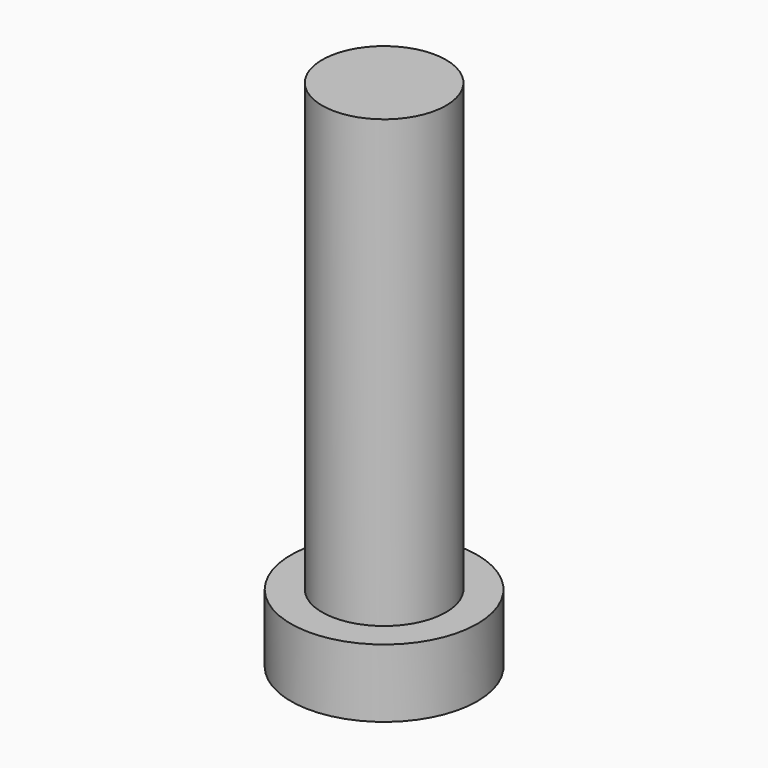
from build123d import *

# Parameters (mm, degrees)
F0_R         = 2
F1_DEPTH     = 14.4
F2_R         = 3.01
F2_R_2       = 2
F3_DEPTH     = 2.2
F4_TEXT_SIZE = 5.2425298943
F5_DEPTH     = 0.2


# Not quite as in the source:
# - Text() gives the source's letters only with a copy of the font that has no kerning and outlines rounded to 1/6400 em; it was checked with that copy


with BuildPart() as f1:
    # F0 (on Top) → F1 (new body)
    with BuildSketch(Plane.XY):
        Circle(F0_R)
    extrude(amount=F1_DEPTH)

    # F2 (on face) → F3 (join)
    with BuildSketch(Plane(origin=(0, 0, 0), x_dir=(1, 0, 0), z_dir=(0, 0, -1))):
        Circle(F2_R)
        Circle(F2_R_2, mode=Mode.SUBTRACT)
        Circle(F2_R_2)
    extrude(amount=F3_DEPTH)

    # F4 (on face) → F5 (cut)
    with BuildSketch(Plane(origin=(0, 0, -2.2), x_dir=(1, 0, 0), z_dir=(0, 0, -1))):
        with Locations((-1.6929193496, -1.7519374378)):
            Text('E', F4_TEXT_SIZE, font='Tinos', font_style=FontStyle.BOLD, text_align=(TextAlign.LEFT, TextAlign.BOTTOM))
    extrude(amount=-F5_DEPTH, mode=Mode.SUBTRACT)


solid = f1.part
